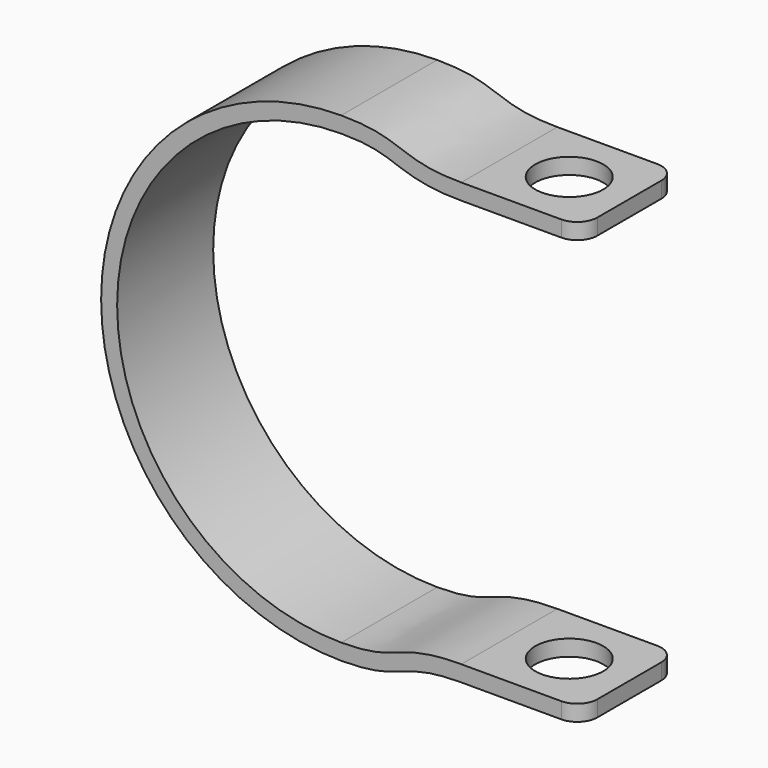
from build123d import *

# Parameters (mm, degrees)
F1_DEPTH = 15
F2_R     = 4.25
F3_DEPTH = 57.5010001
F4_R     = 2.5


with BuildPart() as f1:
    # F0 (on Front) → F1 (new body)
    with BuildSketch(Plane.XZ):
        with BuildLine():
            add(Edge.make_bspline(
                [(0, 30), (4, 30), (7.5, 28.75), (11, 27.5), (15, 27.5)],
                knots=[0, 0, 0, 0, 0.5, 1, 1, 1, 1], degree=3))
            ThreePointArc((0, 30), (-30, 0), (0, -30))
            add(Edge.make_bspline(
                [(0, -30), (4, -30), (7.5, -28.75), (11, -27.5), (15, -27.5)],
                knots=[0, 0, 0, 0, 0.5, 1, 1, 1, 1], degree=3))
            Line((15, -27.5), (30, -27.5))
            Line((30, -27.5), (30, -25.5))
            Line((30, -25.5), (15, -25.5))
            add(Edge.make_bspline(
                [(0, -28), (0.9479166667, -28), (2.545627371, -27.9257628543), (4.2644793503, -27.6643268292), (5.5750060944, -27.3123641034), (6.7972377618, -26.8779672135), (8.2000060944, -26.3748641034), (9.9363543503, -25.9065143292), (12.108127371, -25.5820128543), (13.9479166667, -25.5), (15, -25.5)],
                knots=[0, 0, 0, 0, 0.125, 0.25, 0.375, 0.5, 0.625, 0.75, 0.875, 1, 1, 1, 1], degree=3))
            ThreePointArc((0, -28), (-28, 0), (0, 28))
            add(Edge.make_bspline(
                [(0, 28), (0.9479166667, 28), (2.545627371, 27.9257628543), (4.2644793503, 27.6643268292), (5.5750060944, 27.3123641034), (6.7972377618, 26.8779672135), (8.2000060944, 26.3748641034), (9.9363543503, 25.9065143292), (12.108127371, 25.5820128543), (13.9479166667, 25.5), (15, 25.5)],
                knots=[0, 0, 0, 0, 0.125, 0.25, 0.375, 0.5, 0.625, 0.75, 0.875, 1, 1, 1, 1], degree=3))
            Line((15, 25.5), (30, 25.5))
            Line((30, 25.5), (30, 27.5))
            Line((30, 27.5), (15, 27.5))
        make_face()
    extrude(amount=F1_DEPTH)

    # F2 (on face) → F3 (cut, through all)
    with BuildSketch(Plane.XY.offset(27.5)):
        with Locations((22.5, -7.5)):
            Circle(F2_R)
    extrude(amount=-F3_DEPTH, mode=Mode.SUBTRACT)

    # F4
    f4_edges = [f1.edges().sort_by_distance(p)[0] for p in [
        (30, -15, 26.5),
        (30, -15, -26.5),
        (30, 0, 26.5),
        (30, 0, -26.5),
    ]]
    fillet(f4_edges, radius=F4_R)


solid = f1.part
